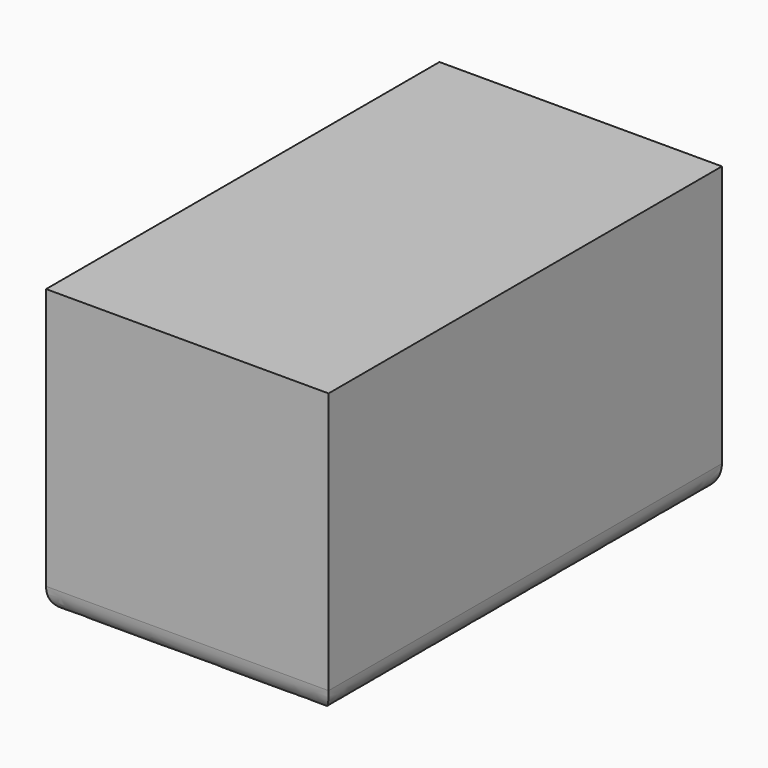
from build123d import *

# Parameters (mm, degrees)
F0_W        = 61.2871013582
F0_H        = 61.8507722393
F1_DEPTH    = 106.68
F2_T1_DEPTH = 132.08
F2_T3_DEPTH = 86.6871013582


# Not quite as in the source:
# - a fillet or chamfer that OpenCascade refuses, or shapes differently, is made with other operations: its cross-section is extruded or revolved along the edge and cut away or added


with BuildPart() as f1:
    # F0 (on Front) → F1 (new body)
    with BuildSketch(Plane.XZ):
        with Locations((-93.0716339499, 26.758744847)):
            Rectangle(F0_W, F0_H)
    extrude(amount=F1_DEPTH)

    # F2: fillet of radius 5.08 on 4 edges, made by hand

    # F2_s2 → F2_t1 (cut)
    with BuildSketch(Plane.XZ.offset(-12.7)):
        with BuildLine():
            add(Edge.make_bspline(
                [(-123.715184629, 0.9133587274), (-123.715184629, -4.1666412726), (-118.635184629, -4.1666412726)],
                knots=[0, 0, 0, 1, 1, 1], degree=2, weights=[1, 1, 1]))
            Line((-118.635184629, -4.1666412726), (-123.715184629, -4.1666412726))
            Line((-123.715184629, -4.1666412726), (-123.715184629, 0.9133587274))
        make_face()
        with BuildLine():
            add(Edge.make_bspline(
                [(-67.5080832708, -4.1666412726), (-62.4280832708, -4.1666412726), (-62.4280832708, 0.9133587274)],
                knots=[0, 0, 0, 1, 1, 1], degree=2, weights=[1, 1, 1]))
            Line((-62.4280832708, 0.9133587274), (-62.4280832708, -4.1666412726))
            Line((-62.4280832708, -4.1666412726), (-67.5080832708, -4.1666412726))
        make_face()
    extrude(amount=F2_T1_DEPTH, mode=Mode.SUBTRACT)

    # F2_s4 → F2_t3 (cut)
    with BuildSketch(Plane.YZ.offset(-136.415184629)):
        with BuildLine():
            add(Edge.make_bspline(
                [(-101.6, -4.1666412726), (-106.68, -4.1666412726), (-106.68, 0.9133587274)],
                knots=[0, 0, 0, 1, 1, 1], degree=2, weights=[1, 1, 1]))
            Line((-106.68, 0.9133587274), (-106.68, -4.1666412726))
            Line((-106.68, -4.1666412726), (-101.6, -4.1666412726))
        make_face()
        with BuildLine():
            add(Edge.make_bspline(
                [(-5.08, -4.1666412726), (0, -4.1666412726), (0, 0.9133587274)],
                knots=[0, 0, 0, 1, 1, 1], degree=2, weights=[1, 1, 1]))
            Line((0, 0.9133587274), (0, -4.1666412726))
            Line((0, -4.1666412726), (-5.08, -4.1666412726))
        make_face()
    extrude(amount=F2_T3_DEPTH, mode=Mode.SUBTRACT)


solid = f1.part
